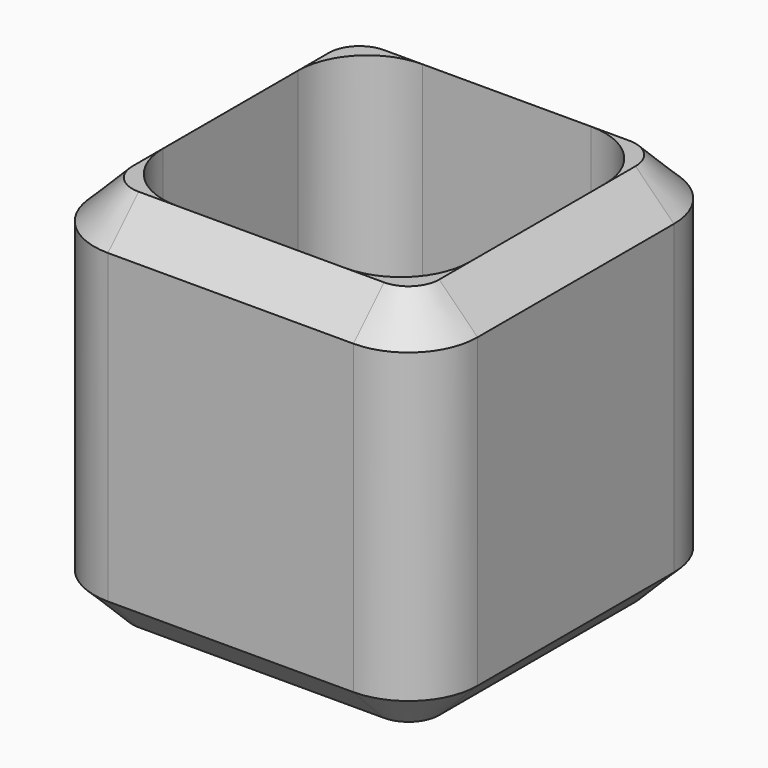
from build123d import *

# Parameters (mm, degrees)
F0_W     = 50
F0_H     = 50
F1_DEPTH = 50
F2_T     = -5
F3_R     = 9
F4_SIZE  = 4.99999


# Not quite as in the source:
# - a fillet or chamfer is up to 0.001 mm smaller than in the source, because OpenCascade refuses the exact size


with BuildPart() as f1:
    # F0 (on Top) → F1 (new body)
    with BuildSketch(Plane.XY):
        Rectangle(F0_W, F0_H)
    extrude(amount=F1_DEPTH)

    # F2
    f2_openings = [f1.faces().sort_by_distance(p)[0] for p in [
        (0, 0, 50),
    ]]
    offset(amount=F2_T, openings=f2_openings)

    # F3
    f3_edges = [f1.edges().sort_by_distance(p)[0] for p in [
        (-25, 25, 25),
        (-25, -25, 25),
        (25, -25, 25),
        (25, 25, 25),
        (20, -20, 27.5),
        (-20, -20, 27.5),
        (-20, 20, 27.5),
        (20, 20, 27.5),
    ]]
    fillet(f3_edges, radius=F3_R)

    # F4 (size 5 in the source; OpenCascade refuses exactly that, so slightly less here)
    f4_edges = [f1.edges().sort_by_distance(p)[0] for p in [
        (25, 0, 0),
        (25, -16, 25),
        (25, 16, 25),
        (25, 0, 50),
        (0, 25, 0),
        (16, 25, 25),
        (-16, 25, 25),
        (0, 25, 50),
        (-25, 0, 0),
        (-25, 16, 25),
        (-25, -16, 25),
        (-25, 0, 50),
        (0, -25, 0),
        (-16, -25, 25),
        (16, -25, 25),
        (0, -25, 50),
    ]]
    chamfer(f4_edges, length=F4_SIZE)


solid = f1.part
